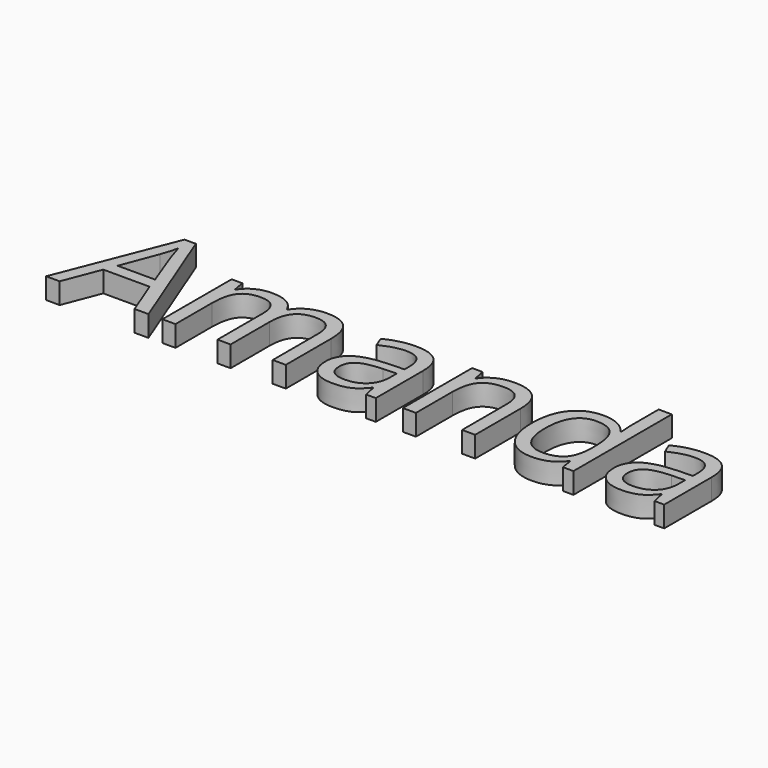
from build123d import *

# Parameters (mm, degrees)
F0_TEXT_SIZE = 39.2214894644
F1_DEPTH     = 5.08


# Not quite as in the source:
# - Text() gives the source's letters only with a copy of the font that has no kerning and outlines rounded to 1/6400 em; it was checked with that copy


with BuildPart() as f1:
    # F0 (on Top) → F1 (new body)
    with BuildSketch(Plane.XY):
        with Locations((-74.0081898928, -13.7009320715)):
            Text('Amanda', F0_TEXT_SIZE, font='Open Sans', text_align=(TextAlign.LEFT, TextAlign.BOTTOM))
    extrude(amount=F1_DEPTH)


solid = f1.part
